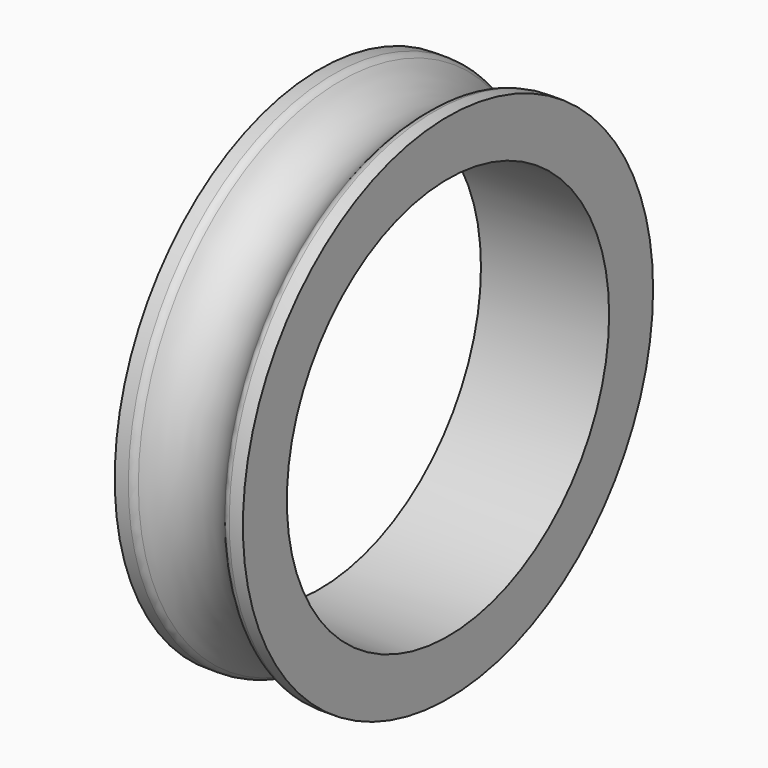
from build123d import *

# Parameters (mm, degrees)
F2_R = 0.5


with BuildPart() as f1:
    # F0 (on Top) → F1 (revolve)
    with BuildSketch(Plane.XY):
        with BuildLine():
            Line((-3.5, -1.5), (3.5, -1.5))
            Line((3.5, -1.5), (3.5, 1.5))
            Line((3.5, 1.5), (2.5, 1.5))
            ThreePointArc((2.5, 1.5), (0, 0.1583123952), (-2.5, 1.5))
            Line((-2.5, 1.5), (-3.5, 1.5))
            Line((-3.5, 1.5), (-3.5, -1.5))
        make_face()
    revolve(axis=Axis((0, -12.5, 0), (1, 0, 0)))

    # F2
    f2_edges = [f1.edges().sort_by_distance(p)[0] for p in [
        (-2.5, -26.5, 0),
        (2.5, -26.5, 0),
    ]]
    fillet(f2_edges, radius=F2_R)


solid = f1.part
